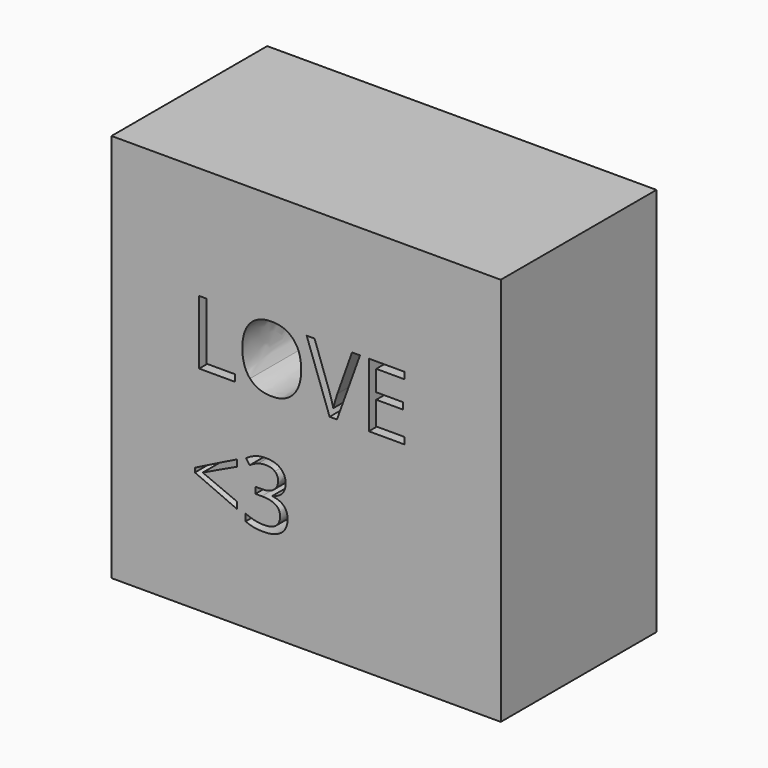
from build123d import *

# Parameters (mm, degrees)
F0_W     = 50.8
F0_H     = 50.8
F1_DEPTH = 25.4


with BuildPart() as f1:
    # F0 (on Front) → F1 (new body)
    with BuildSketch(Plane.XZ):
        with Locations((15.1133043692, 10.5228427142)):
            Rectangle(F0_W, F0_H)
        Polygon((6.0826331481, -0.7500971721), (6.0826331481, -1.6127783157), (0.5940071434, 0.7979768292), (0.5940071434, 1.3572574011), (6.0826331481, 4.0933456892), (6.0826331481, 3.2434585456), (1.61569943, 1.1233099724), align=None, mode=Mode.SUBTRACT)
        with BuildLine():
            add(Edge.make_bspline(
                [(11.7595137243, 4.9185586899), (12.4339402963, 4.3620196894), (12.4339402963, 3.3915034029)],
                knots=[0, 0, 0, 1, 1, 1], degree=2))
            add(Edge.make_bspline(
                [(12.4339402963, 3.3915034029), (12.4339402963, 2.5909645451), (11.9852364388, 2.0828599732)],
                knots=[0, 0, 0, 1, 1, 1], degree=2))
            add(Edge.make_bspline(
                [(11.9852364388, 2.0828599732), (11.5365325813, 1.5747554013), (10.714061152, 1.4029502583)],
                knots=[0, 0, 0, 1, 1, 1], degree=2))
            Line((10.714061152, 1.4029502583), (10.714061152, 1.3572574011))
            add(Edge.make_bspline(
                [(10.714061152, 1.3572574011), (11.71930401, 1.2329728296), (12.2045621533, 0.7184712577)],
                knots=[0, 0, 0, 1, 1, 1], degree=2))
            add(Edge.make_bspline(
                [(12.2045621533, 0.7184712577), (12.6898202965, 0.2039696859), (12.6898202965, -0.6294680291)],
                knots=[0, 0, 0, 1, 1, 1], degree=2))
            add(Edge.make_bspline(
                [(12.6898202965, -0.6294680291), (12.6898202965, -1.8229654587), (11.8618657244, -2.4663208878)],
                knots=[0, 0, 0, 1, 1, 1], degree=2))
            add(Edge.make_bspline(
                [(11.8618657244, -2.4663208878), (11.0339111523, -3.109676317), (9.5095974367, -3.109676317)],
                knots=[0, 0, 0, 1, 1, 1], degree=2))
            add(Edge.make_bspline(
                [(9.5095974367, -3.109676317), (8.8461371504, -3.109676317), (8.2950812928, -3.0091520312)],
                knots=[0, 0, 0, 1, 1, 1], degree=2))
            add(Edge.make_bspline(
                [(8.2950812928, -3.0091520312), (7.7440254352, -2.9086277454), (7.2249545776, -2.658230888)],
                knots=[0, 0, 0, 1, 1, 1], degree=2))
            Line((7.2249545776, -2.658230888), (7.2249545776, -1.7553400301))
            add(Edge.make_bspline(
                [(7.2249545776, -1.7553400301), (7.7677857209, -2.0240140303), (8.3818977214, -2.1638341733)],
                knots=[0, 0, 0, 1, 1, 1], degree=2))
            add(Edge.make_bspline(
                [(8.3818977214, -2.1638341733), (8.996009722, -2.3036543163), (9.5443240081, -2.3036543163)],
                knots=[0, 0, 0, 1, 1, 1], degree=2))
            add(Edge.make_bspline(
                [(9.5443240081, -2.3036543163), (11.7083377243, -2.3036543163), (11.7083377243, -0.6075354577)],
                knots=[0, 0, 0, 1, 1, 1], degree=2))
            add(Edge.make_bspline(
                [(11.7083377243, -0.6075354577), (11.7083377243, 0.9131228293), (9.3213428651, 0.9131228293)],
                knots=[0, 0, 0, 1, 1, 1], degree=2))
            Line((9.3213428651, 0.9131228293), (8.4988714358, 0.9131228293))
            Line((8.4988714358, 0.9131228293), (8.4988714358, 1.7282834015))
            Line((8.4988714358, 1.7282834015), (9.3323091508, 1.7282834015))
            add(Edge.make_bspline(
                [(9.3323091508, 1.7282834015), (10.3083085802, 1.7282834015), (10.879469295, 2.1596239733)],
                knots=[0, 0, 0, 1, 1, 1], degree=2))
            add(Edge.make_bspline(
                [(10.879469295, 2.1596239733), (11.4506300098, 2.5909645451), (11.4506300098, 3.3567768314)],
                knots=[0, 0, 0, 1, 1, 1], degree=2))
            add(Edge.make_bspline(
                [(11.4506300098, 3.3567768314), (11.4506300098, 3.9672334034), (11.0311695808, 4.3163268322)],
                knots=[0, 0, 0, 1, 1, 1], degree=2))
            add(Edge.make_bspline(
                [(11.0311695808, 4.3163268322), (10.6117091519, 4.6654202611), (9.8915897227, 4.6654202611)],
                knots=[0, 0, 0, 1, 1, 1], degree=2))
            add(Edge.make_bspline(
                [(9.8915897227, 4.6654202611), (9.3432754365, 4.6654202611), (8.8580172933, 4.5164615467)],
                knots=[0, 0, 0, 1, 1, 1], degree=2))
            add(Edge.make_bspline(
                [(8.8580172933, 4.5164615467), (8.37275915, 4.3675028323), (7.749508578, 3.9672334034)],
                knots=[0, 0, 0, 1, 1, 1], degree=2))
            Line((7.749508578, 3.9672334034), (7.2706474348, 4.6069334039))
            add(Edge.make_bspline(
                [(7.2706474348, 4.6069334039), (7.7842351495, 5.0126859757), (8.4550062929, 5.243891833)],
                knots=[0, 0, 0, 1, 1, 1], degree=2))
            add(Edge.make_bspline(
                [(8.4550062929, 5.243891833), (9.1257774364, 5.4750976904), (9.8696571513, 5.4750976904)],
                knots=[0, 0, 0, 1, 1, 1], degree=2))
            add(Edge.make_bspline(
                [(9.8696571513, 5.4750976904), (11.0850871523, 5.4750976904), (11.7595137243, 4.9185586899)],
                knots=[0, 0, 0, 1, 1, 1], degree=2))
        make_face(mode=Mode.SUBTRACT)
        Polygon((5.8029928621, 12.9138948396), (1.1478045724, 12.9138948396), (1.1478045724, 21.2647214181), (2.118320859, 21.2647214181), (2.118320859, 13.7930254118), (5.8029928621, 13.7930254118), align=None, mode=Mode.SUBTRACT)
        with BuildLine():
            add(Edge.make_bspline(
                [(13.4574602972, 20.2539954173), (14.4681862981, 19.1116739877), (14.4681862981, 17.1011882717)],
                knots=[0, 0, 0, 1, 1, 1], degree=2))
            add(Edge.make_bspline(
                [(14.4681862981, 17.1011882717), (14.4681862981, 15.0961856986), (13.4538048686, 13.947467269)],
                knots=[0, 0, 0, 1, 1, 1], degree=2))
            add(Edge.make_bspline(
                [(13.4538048686, 13.947467269), (12.4394234392, 12.7987488395), (10.6354694377, 12.7987488395)],
                knots=[0, 0, 0, 1, 1, 1], degree=2))
            add(Edge.make_bspline(
                [(10.6354694377, 12.7987488395), (8.7913057218, 12.7987488395), (7.7888044352, 13.9273624119)],
                knots=[0, 0, 0, 1, 1, 1], degree=2))
            add(Edge.make_bspline(
                [(7.7888044352, 13.9273624119), (6.7863031487, 15.0559759843), (6.7863031487, 17.1121545575)],
                knots=[0, 0, 0, 1, 1, 1], degree=2))
            add(Edge.make_bspline(
                [(6.7863031487, 17.1121545575), (6.7863031487, 19.1518837021), (7.7915460067, 20.2741002744)],
                knots=[0, 0, 0, 1, 1, 1], degree=2))
            add(Edge.make_bspline(
                [(7.7915460067, 20.2741002744), (8.7967888647, 21.3963168468), (10.6464357234, 21.3963168468)],
                knots=[0, 0, 0, 1, 1, 1], degree=2))
            add(Edge.make_bspline(
                [(10.6464357234, 21.3963168468), (12.4467342963, 21.3963168468), (13.4574602972, 20.2539954173)],
                knots=[0, 0, 0, 1, 1, 1], degree=2))
        make_face(mode=Mode.SUBTRACT)
        with BuildLine():
            Line((19.1910000164, 15.8948968421), (21.0991337323, 21.2647214181))
            Line((21.0991337323, 21.2647214181), (22.1427585903, 21.2647214181))
            Line((22.1427585903, 21.2647214181), (19.1343408735, 12.9138948396))
            Line((19.1343408735, 12.9138948396), (18.1747908727, 12.9138948396))
            Line((18.1747908727, 12.9138948396), (15.1809948701, 21.2647214181))
            Line((15.1809948701, 21.2647214181), (16.2099980138, 21.2647214181))
            Line((16.2099980138, 21.2647214181), (18.1290980155, 15.861997985))
            add(Edge.make_bspline(
                [(18.1290980155, 15.861997985), (18.4599143015, 14.9298636984), (18.6536520159, 14.0507331263)],
                knots=[0, 0, 0, 1, 1, 1], degree=2))
            add(Edge.make_bspline(
                [(18.6536520159, 14.0507331263), (18.8601837304, 14.9755565556), (19.1910000164, 15.8948968421)],
                knots=[0, 0, 0, 1, 1, 1], degree=2))
        make_face(mode=Mode.SUBTRACT)
        Polygon((27.9457514524, 13.782059126), (27.9457514524, 12.9138948396), (23.2905631627, 12.9138948396), (23.2905631627, 21.2647214181), (27.9457514524, 21.2647214181), (27.9457514524, 20.4020402746), (24.2610794493, 20.4020402746), (24.2610794493, 17.7116448437), (27.7227703094, 17.7116448437), (27.7227703094, 16.8544468429), (24.2610794493, 16.8544468429), (24.2610794493, 13.782059126), align=None, mode=Mode.SUBTRACT)
    extrude(amount=F1_DEPTH)


solid = f1.part
